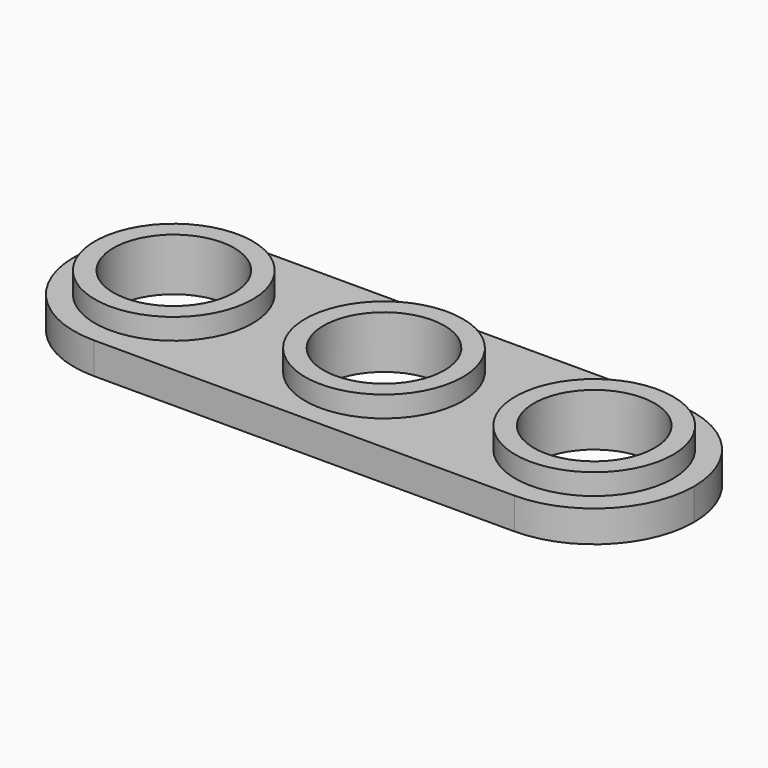
from build123d import *

# Parameters (mm, degrees)
F0_R     = 7.5
F1_DEPTH = 3
F0_R_2   = 5.75
F2_DEPTH = 5


# Not quite as in the source:
# - a feature names something its author has since deleted; it is built from what else it names


with BuildPart() as f1:
    # F0 (on Top) → F1 (new body)
    with BuildSketch(Plane.XY):
        with BuildLine():
            Line((40, 9.5), (0, 9.5))
            ThreePointArc((0, 9.5), (-6.7175144213, 6.7175144213), (-9.5, 0))
            ThreePointArc((-9.5, 0), (-6.7175144213, -6.7175144213), (0, -9.5))
            Line((0, -9.5), (40, -9.5))
            ThreePointArc((40, -9.5), (46.7175144213, -6.7175144213), (49.5, 0))
            ThreePointArc((49.5, 0), (46.7175144213, 6.7175144213), (40, 9.5))
        make_face()
        Circle(F0_R, mode=Mode.SUBTRACT)
        with Locations((20, 0)):
            Circle(F0_R, mode=Mode.SUBTRACT)
        with Locations((40, 0)):
            Circle(F0_R, mode=Mode.SUBTRACT)
    extrude(amount=F1_DEPTH)

    # F0 (on Top) → F2 (join)
    with BuildSketch(Plane.XY):
        Circle(F0_R)
        Circle(F0_R_2, mode=Mode.SUBTRACT)
        with Locations((20, 0)):
            Circle(F0_R)
        with Locations((20, 0)):
            Circle(F0_R_2, mode=Mode.SUBTRACT)
        with Locations((40, 0)):
            Circle(F0_R)
        with Locations((40, 0)):
            Circle(F0_R_2, mode=Mode.SUBTRACT)
    extrude(amount=F2_DEPTH)


solid = f1.part
